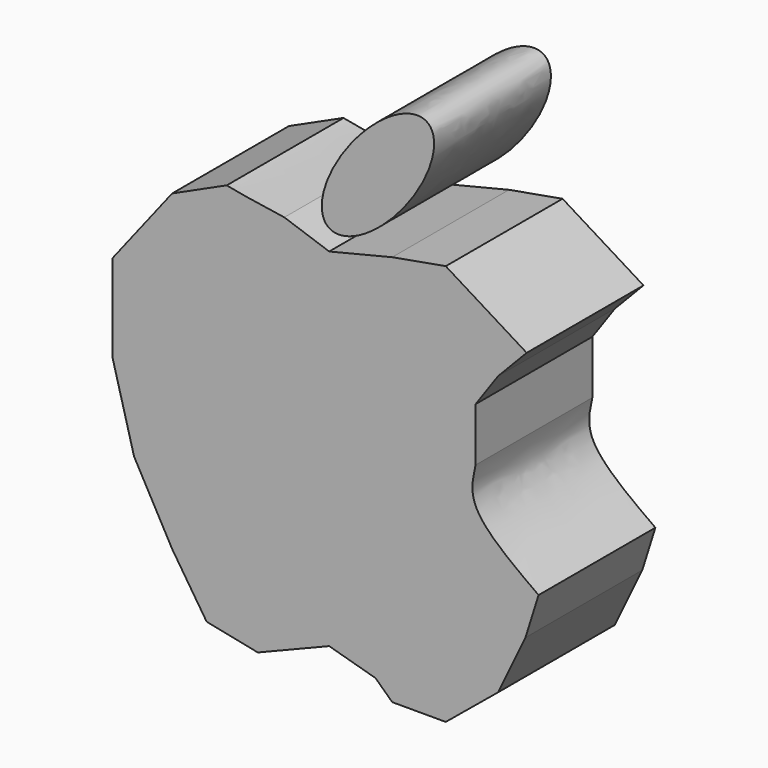
from build123d import *

# Parameters (mm, degrees)
F1_DEPTH = 25.4


with BuildPart() as f1:
    # F0 (on Front) → F1 (new body)
    with BuildSketch(Plane.XZ):
        with BuildLine():
            add(Edge.make_bspline(
                [(42.1581380069, 16.5722500533), (40.5023147662, 14.8474344363), (38.8464915256, 13.1226188193), (37.1906682849, 11.3978032023)],
                knots=[0, 0, 0, 0, 7.1729112397, 7.1729112397, 7.1729112397, 7.1729112397], degree=3))
            add(Edge.make_bspline(
                [(28.0836392194, 25.2653229982), (32.7751388152, 22.3676320165), (37.4666384111, 19.4699410349), (42.1581380069, 16.5722500533)],
                knots=[0, 0, 0, 0, 16.5427033264, 16.5427033264, 16.5427033264, 16.5427033264], degree=3))
            add(Edge.make_bspline(
                [(18.7696348876, 23.6094985157), (21.8743029982, 24.1614400099), (24.9789711088, 24.713381504), (28.0836392194, 25.2653229982)],
                knots=[0, 0, 0, 0, 9.4600439433, 9.4600439433, 9.4600439433, 9.4600439433], degree=3))
            add(Edge.make_bspline(
                [(7.799806539, 20.9187865257), (11.4564159885, 21.8156905224), (15.113025438, 22.7125945191), (18.7696348876, 23.6094985157)],
                knots=[0, 0, 0, 0, 11.2950017712, 11.2950017712, 11.2950017712, 11.2950017712], degree=3))
            add(Edge.make_bspline(
                [(0, 23.6094985157), (2.599935513, 22.7125945191), (5.199871026, 21.8156905224), (7.799806539, 20.9187865257)],
                knots=[0, 0, 0, 0, 8.2508734725, 8.2508734725, 8.2508734725, 8.2508734725], degree=3))
            add(Edge.make_bspline(
                [(-10.0002922118, 25.2653229982), (-10.0127435496, 25.1139003258), (-5.0063717748, 24.3616994208), (0, 23.6094985157)],
                knots=[0.274345513, 0.274345513, 0.274345513, 0.274345513, 1, 1, 1, 1], degree=3))
            add(Edge.make_bspline(
                [(-19.5212755352, 20.9187865257), (-16.3476144274, 22.3676320165), (-13.1739533196, 23.8164775074), (-10.0002922118, 25.2653229982)],
                knots=[0, 0, 0, 0, 10.4662076585, 10.4662076585, 10.4662076585, 10.4662076585], degree=3))
            add(Edge.make_bspline(
                [(-29.8701692373, 7.6722013764), (-26.4205380032, 12.0877297595), (-22.9709067692, 16.5032581426), (-19.5212755352, 20.9187865257)],
                knots=[0, 0, 0, 0, 16.8098667149, 16.8098667149, 16.8098667149, 16.8098667149], degree=3))
            add(Edge.make_bspline(
                [(-29.8701692373, -7.6441620477), (-29.8701692373, -2.538707573), (-29.8701692373, 2.5667469017), (-29.8701692373, 7.6722013764)],
                knots=[0, 0, 0, 0, 15.3163634241, 15.3163634241, 15.3163634241, 15.3163634241], degree=3))
            add(Edge.make_bspline(
                [(-26.1445678771, -21.5116813779), (-27.3864349971, -16.8891749345), (-28.6283021172, -12.2666684911), (-29.8701692373, -7.6441620477)],
                knots=[0, 0, 0, 0, 14.3592547811, 14.3592547811, 14.3592547811, 14.3592547811], degree=3))
            add(Edge.make_bspline(
                [(-19.5212755352, -33.5163995624), (-21.7290396492, -29.5148268342), (-23.9368037631, -25.513254106), (-26.1445678771, -21.5116813779)],
                knots=[0, 0, 0, 0, 13.7106258112, 13.7106258112, 13.7106258112, 13.7106258112], degree=3))
            add(Edge.make_bspline(
                [(-13.518916443, -42.7073811491), (-15.5197028071, -39.6437206202), (-17.5204891711, -36.5800600913), (-19.5212755352, -33.5163995624)],
                knots=[0, 0, 0, 0, 10.9773611219, 10.9773611219, 10.9773611219, 10.9773611219], degree=3))
            add(Edge.make_bspline(
                [(-4.6188673005, -44.5311143994), (-7.585550348, -43.923203316), (-10.5522333955, -43.3152922326), (-13.518916443, -42.7073811491)],
                knots=[0, 0, 0, 0, 9.0849808865, 9.0849808865, 9.0849808865, 9.0849808865], degree=3))
            add(Edge.make_bspline(
                [(7.799806539, -39.5187586546), (3.6602485925, -41.1895439029), (-0.479309354, -42.8603291512), (-4.6188673005, -44.5311143994)],
                knots=[0, 0, 0, 0, 13.3920562291, 13.3920562291, 13.3920562291, 13.3920562291], degree=3))
            add(Edge.make_bspline(
                [(15.8719439059, -41.795514524), (13.1812314503, -41.0365959009), (10.4905189946, -40.2776772777), (7.799806539, -39.5187586546)],
                knots=[0, 0, 0, 0, 8.3870745174, 8.3870745174, 8.3870745174, 8.3870745174], degree=3))
            add(Edge.make_bspline(
                [(18.7696348876, -44.5311143994), (17.8037378937, -43.6192477743), (16.8378408998, -42.7073811491), (15.8719439059, -41.795514524)],
                knots=[0, 0, 0, 0, 3.9849867884, 3.9849867884, 3.9849867884, 3.9849867884], degree=3))
            add(Edge.make_bspline(
                [(28.0836392194, -44.5311143994), (24.9789711088, -44.5311143994), (21.8743029982, -44.5311143994), (18.7696348876, -44.5311143994)],
                knots=[0, 0, 0, 0, 9.3140043318, 9.3140043318, 9.3140043318, 9.3140043318], degree=3))
            add(Edge.make_bspline(
                [(37.1906682849, -37.0350219309), (34.1549919297, -39.5337194204), (31.1193155746, -42.0324169099), (28.0836392194, -44.5311143994)],
                knots=[0, 0, 0, 0, 11.79531181, 11.79531181, 11.79531181, 11.79531181], degree=3))
            add(Edge.make_bspline(
                [(41.9511571527, -27.1000843495), (40.3643275301, -30.41173021), (38.7774979075, -33.7233760705), (37.1906682849, -37.0350219309)],
                knots=[0, 0, 0, 0, 11.0165892638, 11.0165892638, 11.0165892638, 11.0165892638], degree=3))
            add(Edge.make_bspline(
                [(44.2279167473, -19.8558587581), (43.4689968824, -22.2706006219), (42.7100770175, -24.6853424857), (41.9511571527, -27.1000843495)],
                knots=[0, 0, 0, 0, 7.5935787789, 7.5935787789, 7.5935787789, 7.5935787789], degree=3))
            add(Edge.make_bspline(
                [(33.2580842078, -3.5046045668), (32.796057697, -5.55288587), (31.6173669123, -10.7783225931), (39.4596647515, -16.4234961329), (44.2279167473, -19.8558587581)],
                knots=[0, 0, 0, 0, 0.3919827972, 1, 1, 1, 1], degree=3))
            add(Edge.make_bspline(
                [(33.2580842078, -3.5046045668), (33.2580842078, -0.3999361458), (33.2580842078, 2.7047322753), (33.2580842078, 5.8094006963)],
                knots=[0, 0, 0, 0, 9.3140052631, 9.3140052631, 9.3140052631, 9.3140052631], degree=3))
            add(Edge.make_bspline(
                [(37.1906682849, 11.3978032023), (35.8798069259, 9.535002367), (34.5689455668, 7.6722015316), (33.2580842078, 5.8094006963)],
                knots=[0, 0, 0, 0, 6.8334076486, 6.8334076486, 6.8334076486, 6.8334076486], degree=3))
        make_face()
    extrude(amount=F1_DEPTH)


with BuildPart() as f1b:
    # F0 (on Front) → F1, piece 2 (new body)
    with BuildSketch(Plane.XZ):
        with BuildLine():
            add(Edge.make_bspline(
                [(24.9789711088, 46.1700893939), (17.2604187779, 52.4043037105), (8.08008832, 33.1429190243), (-1.1002421379, 13.881534338), (15.7986406509, 26.9087047076), (32.6975234397, 39.9358750772), (24.9789711088, 46.1700893939)],
                knots=[0, 0, 0, 2.0943951024, 2.0943951024, 4.1887902048, 4.1887902048, 6.2831853072, 6.2831853072, 6.2831853072], degree=2, weights=[1, 0.5, 1, 0.5, 1, 0.5, 1]))
        make_face()
    extrude(amount=F1_DEPTH)


solid = Compound([f1.part, f1b.part])
